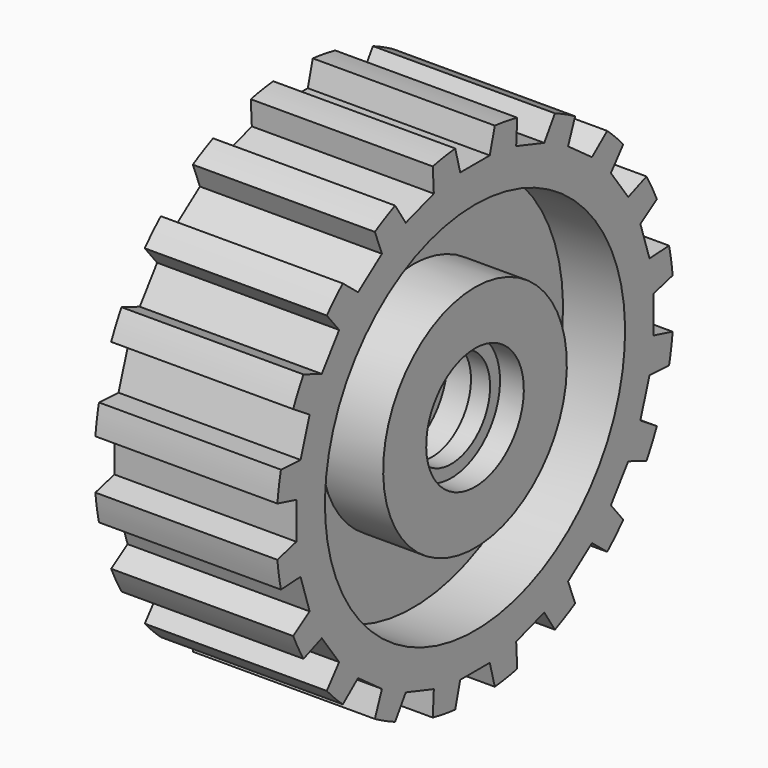
from build123d import *

# Parameters (mm, degrees)
F3_DEPTH        = 88.646
F3_COPIES_COUNT = 20


# Not quite as in the source:
# - a feature of the source that left no trace in its solid (it failed there, or was rolled back) is left out
# - a pattern or mirror of a feature is missing from the dataset's text; its kind, count and spacing are read off the source's solid


with BuildPart() as f1:
    # F0 (on Front) → F1 (revolve)
    with BuildSketch(Plane.XZ):
        Polygon((38.1, 36.1084090909), (38.1, 61.5084090909), (-38.1, 61.5084090909), (-38.1, 36.1084090909), (-11.9062505468, 36.1084090909), (-11.9062505468, 5.6284090909), (-38.1, 5.6284090909), (-38.1, -16.8852278195), (-30.0903403623, -16.8852278195), (-30.0903403623, -21.6477272727), (-22.9465920027, -21.6477272727), (-22.9465920027, -16.8852278195), (-6.0613630896, -16.8852278195), (-6.0613630896, -28.3585221805), (6.0613652768, -28.3585221805), (6.0613652768, -16.8852278195), (20.1323869104, -16.8852278195), (20.1323869104, -22.0806807246), (28.1420443609, -22.0806807246), (28.1420443609, -16.8852278195), (38.1, -16.8852278195), (38.1, 5.6284090909), (12.1227261791, 5.6284090909), (12.1227261791, 36.1084090909), align=None)
    revolve(axis=Axis((0.8659090909, 0, -42.4295432673), (1, 0, 0)))

    # F2 (on face) → F3 (cut, symmetric)
    with BuildSketch(Plane.YZ.offset(28.1420443609)):
        Polygon((0, 65.8745542169), (-11.6578890011, 65.8745542169), (-7.7292122878, 51.0664619505), (0, 51.0664619505), (7.7292122878, 51.0664619505), (11.6578890011, 65.8745542169), align=None)
    f3 = extrude(amount=F3_DEPTH, both=True, mode=Mode.SUBTRACT)

    # F3_copies: F3 ×20 about axis
    f3_copies_axis = Axis((0, 0, -42.429543), (1, 0, 0))
    for i in range(1, F3_COPIES_COUNT):
        add(f3.rotate(f3_copies_axis, i * 360 / F3_COPIES_COUNT), mode=Mode.SUBTRACT)


solid = f1.part
